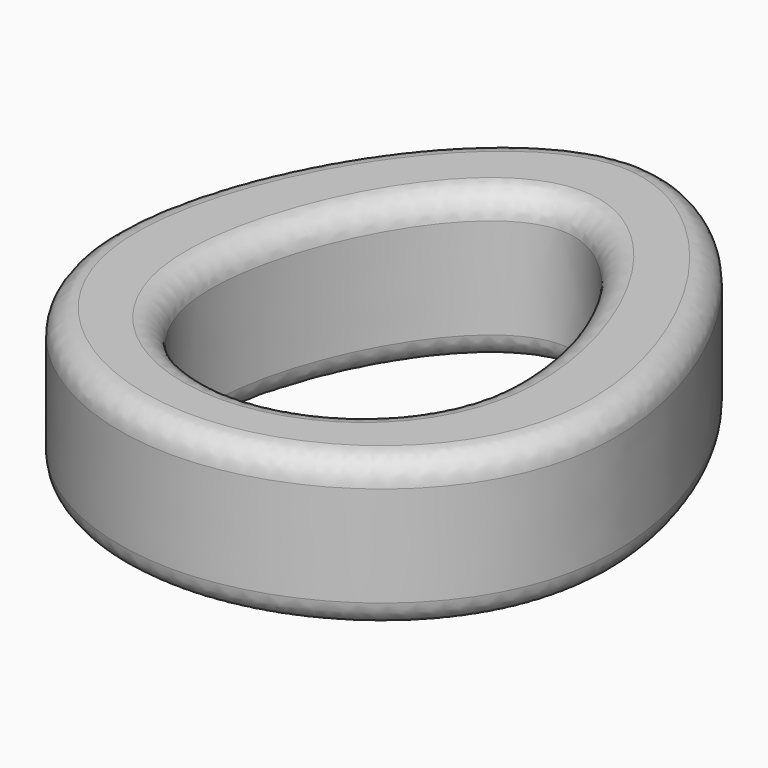
from build123d import *

# Parameters (mm, degrees)
F1_DEPTH = 3
F2_R     = 0.5


with BuildPart() as f1:
    # F0 (on Top) → F1 (new body)
    with BuildSketch(Plane.XY):
        with BuildLine():
            add(Edge.make_bspline(
                [(0, 7.3593744678), (2.6332609756, 7.3593744678), (7.5367444489, -0.662256585), (0, -6.0253556597), (-7.5367444489, -0.662256585), (-2.6332609756, 7.3593744678), (0, 7.3593744678)],
                knots=[0, 0, 0, 0, 0.2685092129, 0.5, 0.7314907871, 1, 1, 1, 1], degree=3))
        make_face()
        with BuildLine():
            add(Edge.make_bspline(
                [(0, 5.3593744678), (1.6198338531, 5.3593744678), (4.5463354891, -0.5248682612), (0, -3.5853001664), (-4.5463354891, -0.5248682612), (-1.6198338531, 5.3593744678), (0, 5.3593744678)],
                knots=[0, 0, 0, 0, 0.2767525966, 0.5, 0.7232474034, 1, 1, 1, 1], degree=3))
        make_face(mode=Mode.SUBTRACT)
    extrude(amount=F1_DEPTH)

    # F2
    f2_edges = [f1.edges().sort_by_distance(p)[0] for p in [
        (0, -4.328126, 0),
        (0, -4.328126, 3),
        (0, -2.640626, 3),
        (0, -2.640626, 0),
    ]]
    fillet(f2_edges, radius=F2_R)


solid = f1.part
